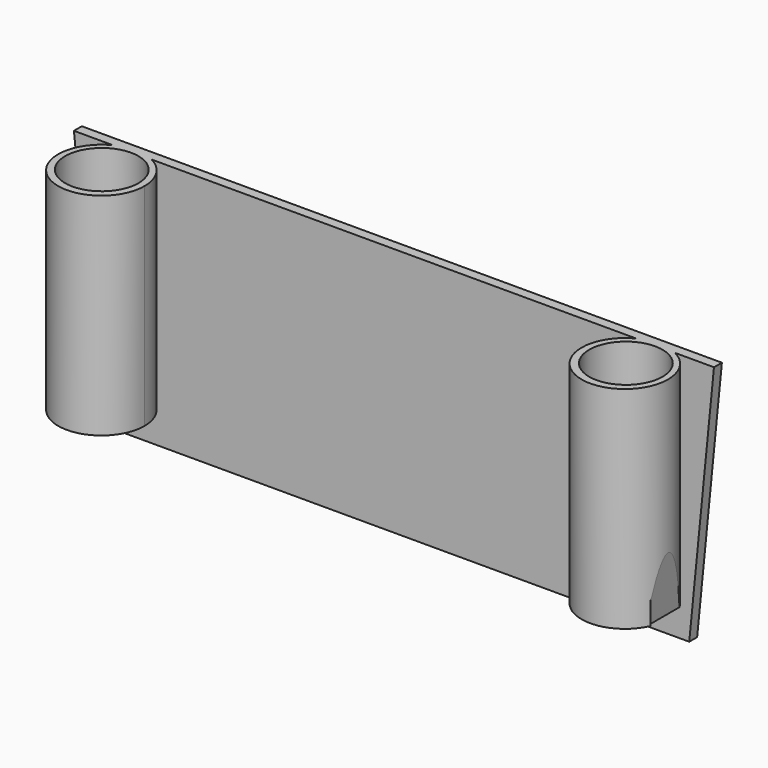
from build123d import *

# Parameters (mm, degrees)
F0_W     = 246.3848441839
F0_H     = 96.1289182305
F1_DEPTH = 3.81
F2_R     = 14.1092662394
F3_DEPTH = 81.28
F5_DEPTH = 25.4
F6_R     = 14.1092662394
F7_DEPTH = 7.62


# Not quite as in the source:
# - a pattern or mirror of a feature is missing from the dataset's text; its kind, count and spacing are read off the source's solid
# - a feature names something its author has since deleted; it is built from what else it names


with BuildPart() as f1:
    # F0 (on Front) → F1 (new body)
    with BuildSketch(Plane.XZ):
        Rectangle(F0_W, F0_H)
    extrude(amount=F1_DEPTH)

    # F2 (on face) → F3 (join)
    with BuildSketch(Plane.XY.offset(48.0644591153)):
        with BuildLine():
            ThreePointArc((-108.1859269769, -3.81), (-109.4788428986, -32.8031453268), (-84.1323126967, -18.6671093106))
            ThreePointArc((-84.1323126967, -18.6671093106), (-86.6114524229, -9.9357548511), (-93.3090499012, -3.81))
            Line((-93.3090499012, -3.81), (-108.1859269769, -3.81))
        make_face()
        with Locations((-100.8657291532, -18.3125622571)):
            Circle(F2_R, mode=Mode.SUBTRACT)
    f3 = extrude(amount=-F3_DEPTH)

    # F3_copies: F3 across plane
    add(f3.mirror(Plane(origin=(0, 0, 0), x_dir=(0, 0, 1), z_dir=(1, 0, 0))))

    # F4 (on face) → F5 (cut)
    with BuildSketch(Plane(origin=(0, 0, 0), x_dir=(-1, 0, 0), z_dir=(0, 1, 0))):
        Polygon((-113.6597358778, -48.0644591153), (-123.1800099188, 48.0619171371), (-123.192422092, 47.8396813394), (-123.192422092, -48.0644591153), align=None)
    f5 = extrude(amount=-F5_DEPTH, mode=Mode.SUBTRACT)

    # F5_copies: F5 across plane
    add(f5.mirror(Plane(origin=(0, 0, 0), x_dir=(0, 0, -1), z_dir=(-1, 0, 0))), mode=Mode.SUBTRACT)

    # F6 (on face) → F7 (join)
    with BuildSketch(Plane(origin=(0, 0, -33.2155408847), x_dir=(1, 0, 0), z_dir=(0, 0, -1))):
        with BuildLine():
            ThreePointArc((-115.130360032, 15.9625050025), (-99.772384803, 3.8619408749), (-86.5015784629, 18.2207971811))
            ThreePointArc((-86.5015784629, 18.2207971811), (-99.772384803, 32.5796534874), (-115.130360032, 20.4790893598))
            Line((-115.130360032, 20.4790893598), (-115.130360032, 15.9625050025))
        make_face()
        with Locations((-100.8657291532, 18.3125622571)):
            Circle(F6_R, mode=Mode.SUBTRACT)
        with Locations((-100.8657291532, 18.3125622571)):
            Circle(F6_R)
    f7 = extrude(amount=-F7_DEPTH)

    # F7_copies: F7 across plane
    add(f7.mirror(Plane(origin=(0, 0, 0), x_dir=(0, 0, 1), z_dir=(1, 0, 0))))


solid = f1.part
